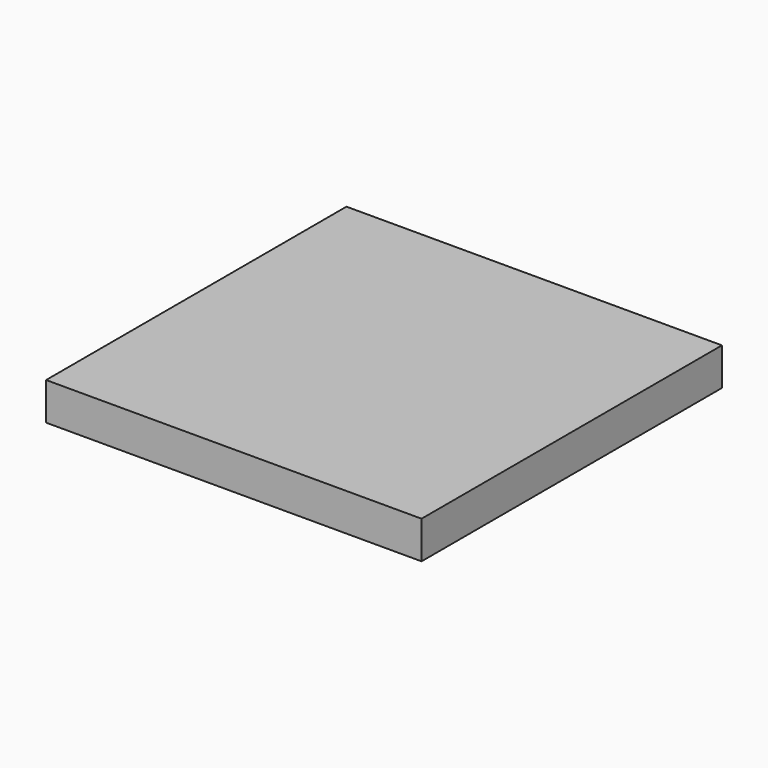
from build123d import *

# Parameters (mm, degrees)
F0_W     = 1000
F0_H     = 1000
F1_DEPTH = 100
F4_DEPTH = 80
F5_DEPTH = 80


# Not quite as in the source:
# - the program builds the solid bodies; features that only make, move or delete a surface that nothing else refers to are left out


with BuildPart() as f1:
    # F0 (on Top) → F1 (new body)
    with BuildSketch(Plane.XY):
        with Locations((-0.4372149706, 133.5517169366)):
            Rectangle(F0_W, F0_H)
    extrude(amount=F1_DEPTH)

    # F2 (on Top) → F4 (cut)
    with BuildSketch(Plane.XY):
        Polygon((66.5457851066, 298.988878727), (-66.5457851066, 298.988878727), (-160.6557369232, 204.8789269104), (-160.6557369232, 71.7873566971), (-66.5457851066, -22.3225951195), (66.5457851066, -22.3225951195), (160.6557369232, 71.7873566971), (160.6557369232, 204.8789269104), align=None)
    extrude(amount=F4_DEPTH, mode=Mode.SUBTRACT)

    # F5 (add): a face of the model
    f5_faces = [f1.faces().sort_by_distance(p)[0] for p in [
        (0, 138.3331418037, 80),
    ]]
    extrude(f5_faces, amount=F5_DEPTH)


solid = f1.part
